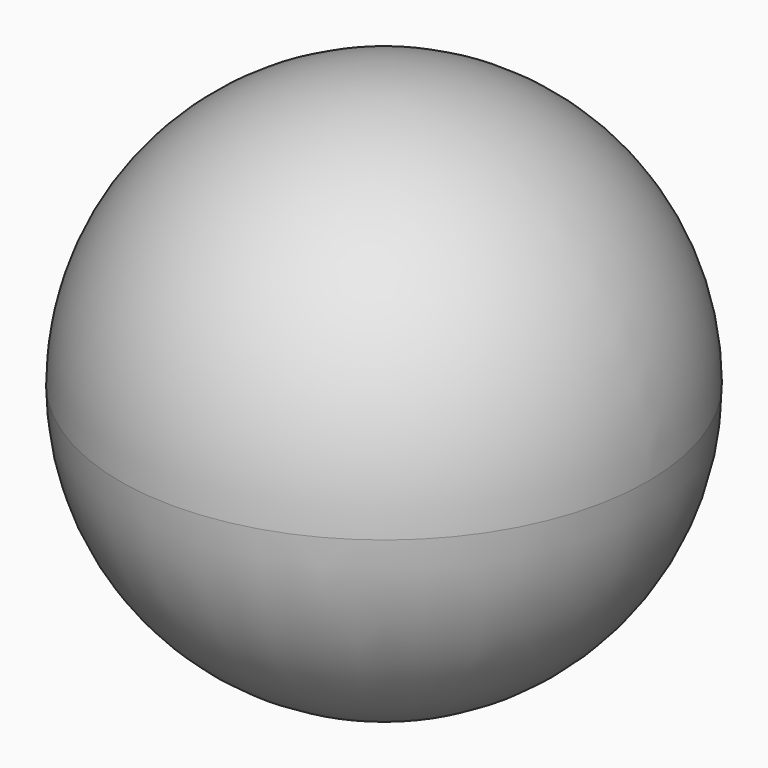
from build123d import *

# Parameters (mm, degrees)
F0_R     = 7.5
F1_DEPTH = 7.5
F2_R     = 7.5
F3_R     = 7.49999


# Not quite as in the source:
# - a fillet or chamfer is up to 0.001 mm smaller than in the source, because OpenCascade refuses the exact size


with BuildPart() as f1:
    # F0 (on Top) → F1 (new body, symmetric)
    with BuildSketch(Plane.XY):
        Circle(F0_R)
    extrude(amount=F1_DEPTH, both=True)

    # F2
    f2_edges = [f1.edges().sort_by_distance(p)[0] for p in [
        (-7.5, 0, 7.5),
    ]]
    fillet(f2_edges, radius=F2_R)

    # F3 (radius 7.5 in the source; OpenCascade refuses exactly that, so slightly less here)
    f3_edges = [f1.edges().sort_by_distance(p)[0] for p in [
        (-7.5, 0, -7.5),
    ]]
    fillet(f3_edges, radius=F3_R)


solid = f1.part
